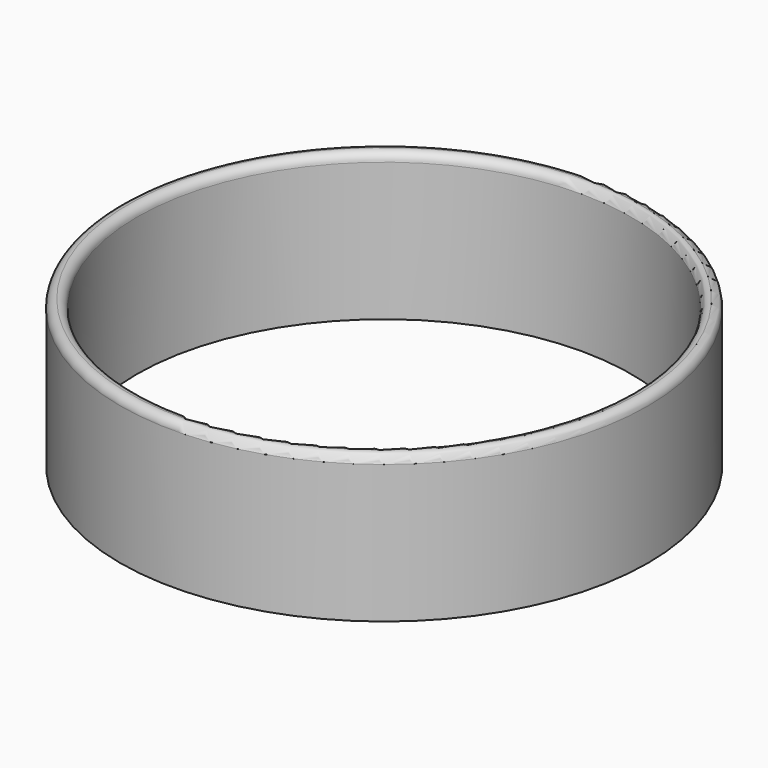
from build123d import *

# Parameters (mm, degrees)
F0_R     = 63
F0_R_2   = 59
F1_DEPTH = 35
F2_R     = 1.99999


# Not quite as in the source:
# - a fillet or chamfer is up to 0.001 mm smaller than in the source, because OpenCascade refuses the exact size


with BuildPart() as f1:
    # F0 (on Top) → F1 (new body)
    with BuildSketch(Plane.XY):
        Circle(F0_R)
        Circle(F0_R_2, mode=Mode.SUBTRACT)
    extrude(amount=F1_DEPTH)

    # F2 (radius 2 in the source; OpenCascade refuses exactly that, so slightly less here)
    f2_edges = [f1.edges().sort_by_distance(p)[0] for p in [
        (-59, 0, 35),
        (-63, 0, 35),
    ]]
    fillet(f2_edges, radius=F2_R)


solid = f1.part
